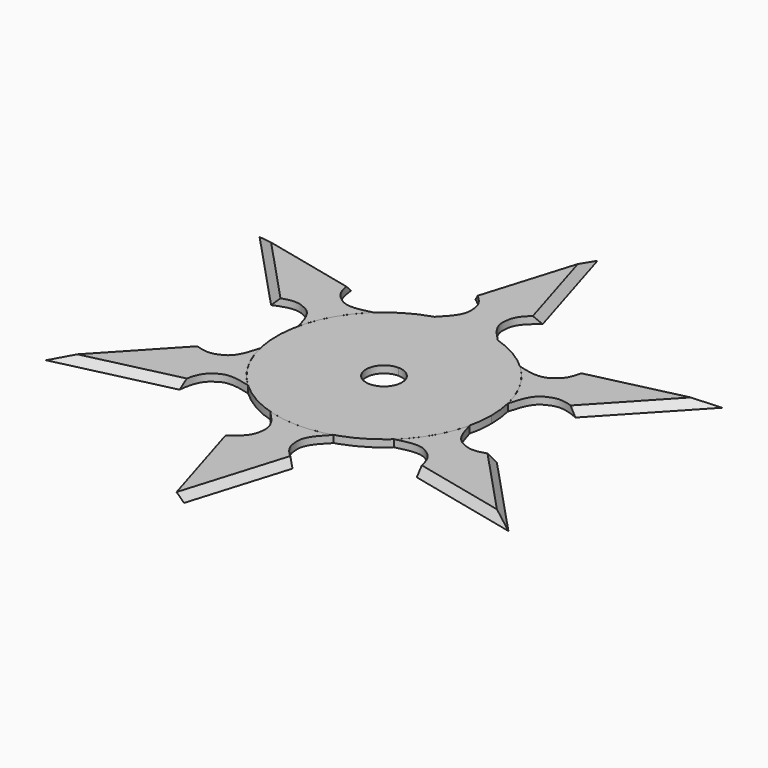
from build123d import *

# Parameters (mm, degrees)
F1_DEPTH      = 1.27
F2_COUNT      = 6
F3_DEPTH      = 1.27
F4_T1_DEPTH   = 28.2648616639
F4_T3_DEPTH   = 28.2648616639
F4_2_T1_DEPTH = 28.2648616639
F4_2_T3_DEPTH = 28.2648616639
F4_3_T1_DEPTH = 28.2648616639
F4_3_T3_DEPTH = 28.2648616639
F4_4_T1_DEPTH = 28.2648616639
F4_4_T3_DEPTH = 28.2648616639
F4_5_T1_DEPTH = 28.2648616639
F4_5_T3_DEPTH = 28.2648616639
F4_6_T1_DEPTH = 28.2648616639
F4_6_T3_DEPTH = 28.2648616639


# Not quite as in the source:
# - a fillet or chamfer that OpenCascade refuses, or shapes differently, is made with other operations: its cross-section is extruded or revolved along the edge and cut away or added


with BuildPart() as f1:
    # F0 (on Top) → F1 (new body)
    with BuildSketch(Plane.XY):
        Polygon((0, 27.8319306672), (6.0893329792, 27.8319306672), (0, 47.8763319552), align=None)
        Polygon((0, 47.8763319552), (-6.0893329792, 27.8319306672), (0, 27.8319306672), align=None)
        with BuildLine():
            add(Edge.make_bspline(
                [(-5.6085209245, 18.2056857338), (-2.7667914864, 20.9939918215), (-2.759898495, 23.1821026248), (-3.1363011766, 25.7094376402), (-6.0893329792, 27.8319306672)],
                knots=[0, 0, 0, 0, 0.5044710626, 1, 1, 1, 1], degree=3))
            ThreePointArc((-5.6085209245, 18.2056857338), (-2.8358584917, 18.8377388934), (0, 19.05))
            Line((0, 19.05), (0, 27.8319306672))
            Line((0, 27.8319306672), (-6.0893329792, 27.8319306672))
        make_face()
        with BuildLine():
            ThreePointArc((0, 19.05), (2.8358584917, 18.8377388934), (5.6085209245, 18.2056857338))
            add(Edge.make_bspline(
                [(5.6085209245, 18.2056857338), (2.7667914864, 20.9939918215), (2.759898495, 23.1821026248), (3.1363011766, 25.7094376402), (6.0893329792, 27.8319306672)],
                knots=[0, 0, 0, 0, 0.5044710626, 1, 1, 1, 1], degree=3))
            Line((6.0893329792, 27.8319306672), (0, 27.8319306672))
            Line((0, 27.8319306672), (0, 19.05))
        make_face()
    extrude(amount=F1_DEPTH)


with BuildPart() as f2_1:
    # F2: instance of F1
    add(f1.part.rotate(Axis((0, 0, 0), (0, 0, 1)), 1 * 360 / F2_COUNT))

    # F4#2: chamfer of 1.4224 on 2 edges, made by hand

    # F4_2_s2 → F4_2_t1 (cut)
    with BuildSketch(Plane(origin=(-20.6503164596, 4.8060973638, 0), x_dir=(0, 0, 1), z_dir=(-0.9739695304, 0.2266789665, 0))):
        Polygon((-0.1524, 13.9164538313), (1.27, 12.4940538313), (1.27, 13.9164538313), align=None)
    extrude(amount=F4_2_T1_DEPTH, mode=Mode.SUBTRACT)

    # F4_2_s4 → F4_2_t3 (cut)
    with BuildSketch(Plane(origin=(-33.8005854034, 36.1180372572, 0), x_dir=(0, 0, 1), z_dir=(0.6832945087, -0.7301428726, 0))):
        Polygon((-0.1524, 13.9164538313), (1.27, 12.4940538313), (1.27, 13.9164538313), align=None)
    extrude(amount=F4_2_T3_DEPTH, mode=Mode.SUBTRACT)


with BuildPart() as f2_2:
    # F2: instance of F1
    add(f1.part.rotate(Axis((0, 0, 0), (0, 0, 1)), 2 * 360 / F2_COUNT))

    # F4#3: chamfer of 1.4224 on 2 edges, made by hand

    # F4_3_s2 → F4_3_t1 (cut)
    with BuildSketch(Plane(origin=(-48.1794305013, -11.2131469935, 0), x_dir=(0, 0, 1), z_dir=(0.9739695304, 0.2266789665, 0))):
        Polygon((-0.1524, 13.9164538313), (1.27, 12.4940538313), (1.27, 13.9164538313), align=None)
    extrude(amount=F4_3_T1_DEPTH, mode=Mode.SUBTRACT)

    # F4_3_s4 → F4_3_t3 (cut)
    with BuildSketch(Plane(origin=(-14.4873606399, -15.4806499682, 0), x_dir=(0, 0, 1), z_dir=(-0.6832945087, -0.7301428726, 0))):
        Polygon((-0.1524, 13.9164538313), (1.27, 12.4940538313), (1.27, 13.9164538313), align=None)
    extrude(amount=F4_3_T3_DEPTH, mode=Mode.SUBTRACT)


with BuildPart() as f2_3:
    # F2: instance of F1
    add(f1.part.rotate(Axis((0, 0, 0), (0, 0, 1)), 3 * 360 / F2_COUNT))

    # F4#4: chamfer of 1.4224 on 2 edges, made by hand

    # F4_4_s2 → F4_4_t1 (cut)
    with BuildSketch(Plane(origin=(-14.3788450979, -47.3311842507, 0), x_dir=(0, 0, 1), z_dir=(0.2906750217, 0.9568218391, 0))):
        Polygon((-0.1524, 13.9164538313), (1.27, 12.4940538313), (1.27, 13.9164538313), align=None)
    extrude(amount=F4_4_T1_DEPTH, mode=Mode.SUBTRACT)

    # F4_4_s4 → F4_4_t3 (cut)
    with BuildSketch(Plane(origin=(6.1629558196, -20.2867473321, 0), x_dir=(0, 0, 1), z_dir=(0.2906750217, -0.9568218391, 0))):
        Polygon((1.4224, 13.9164538313), (0, 12.4940538313), (0, 13.9164538313), align=None)
    extrude(amount=F4_4_T3_DEPTH, mode=Mode.SUBTRACT)


with BuildPart() as f2_4:
    # F2: instance of F1
    add(f1.part.rotate(Axis((0, 0, 0), (0, 0, 1)), 4 * 360 / F2_COUNT))

    # F4#5: chamfer of 1.4224 on 2 edges, made by hand

    # F4_5_s2 → F4_5_t1 (cut)
    with BuildSketch(Plane(origin=(33.8005854034, -36.1180372572, 0), x_dir=(0, 0, 1), z_dir=(-0.6832945087, 0.7301428726, 0))):
        Polygon((-0.1524, 13.9164538313), (1.27, 12.4940538313), (1.27, 13.9164538313), align=None)
    extrude(amount=F4_5_T1_DEPTH, mode=Mode.SUBTRACT)

    # F4_5_s4 → F4_5_t3 (cut)
    with BuildSketch(Plane(origin=(20.6503164596, -4.8060973638, 0), x_dir=(0, 0, 1), z_dir=(0.9739695304, -0.2266789665, 0))):
        Polygon((-0.1524, 13.9164538313), (1.27, 12.4940538313), (1.27, 13.9164538313), align=None)
    extrude(amount=F4_5_T3_DEPTH, mode=Mode.SUBTRACT)


with BuildPart() as f2_5:
    # F2: instance of F1
    add(f1.part.rotate(Axis((0, 0, 0), (0, 0, 1)), 5 * 360 / F2_COUNT))

    # F4#6: chamfer of 1.4224 on 2 edges, made by hand

    # F4_6_s2 → F4_6_t1 (cut)
    with BuildSketch(Plane(origin=(48.1794305013, 11.2131469935, 0), x_dir=(0, 0, 1), z_dir=(-0.9739695304, -0.2266789665, 0))):
        Polygon((-0.1524, 13.9164538313), (1.27, 12.4940538313), (1.27, 13.9164538313), align=None)
    extrude(amount=F4_6_T1_DEPTH, mode=Mode.SUBTRACT)

    # F4_6_s4 → F4_6_t3 (cut)
    with BuildSketch(Plane(origin=(14.4873606399, 15.4806499682, 0), x_dir=(0, 0, 1), z_dir=(0.6832945087, 0.7301428726, 0))):
        Polygon((-0.1524, 13.9164538313), (1.27, 12.4940538313), (1.27, 13.9164538313), align=None)
    extrude(amount=F4_6_T3_DEPTH, mode=Mode.SUBTRACT)


with BuildPart() as f1_1:
    add(f1.part)

    # F0 (on Top) → F3 (join)
    with BuildSketch(Plane.XY):
        with BuildLine():
            ThreePointArc((-5.6085209245, 18.2056857338), (-11.3150381437, -15.3255476837), (19.05, 0))
            ThreePointArc((19.05, 0), (15.3255476837, 11.3150381437), (5.6085209245, 18.2056857338))
            ThreePointArc((5.6085209245, 18.2056857338), (2.8358584917, 18.8377388934), (0, 19.05))
            ThreePointArc((0, 19.05), (-2.8358584917, 18.8377388934), (-5.6085209245, 18.2056857338))
        make_face()
        with BuildLine():
            ThreePointArc((3.175, 0), (-2.2450640303, -2.2450640303), (0, 3.175))
            ThreePointArc((0, 3.175), (2.2450640303, 2.2450640303), (3.175, 0))
        make_face(mode=Mode.SUBTRACT)
    extrude(amount=F3_DEPTH)

    # F4: chamfer of 1.4224 on 2 edges, made by hand

    # F4_s2 → F4_t1 (cut)
    with BuildSketch(Plane(origin=(14.3788450979, 47.3311842507, 0), x_dir=(0, 0, 1), z_dir=(-0.2906750217, -0.9568218391, 0))):
        Polygon((-0.1524, 13.9164538313), (1.27, 12.4940538313), (1.27, 13.9164538313), align=None)
    extrude(amount=F4_T1_DEPTH, mode=Mode.SUBTRACT)

    # F4_s4 → F4_t3 (cut)
    with BuildSketch(Plane(origin=(-6.1629558196, 20.2867473321, 0), x_dir=(0, 0, 1), z_dir=(-0.2906750217, 0.9568218391, 0))):
        Polygon((-0.1524, 13.9164538313), (1.27, 12.4940538313), (1.27, 13.9164538313), align=None)
    extrude(amount=F4_T3_DEPTH, mode=Mode.SUBTRACT)


solid = Compound([f2_1.part, f2_2.part, f2_3.part, f2_4.part, f2_5.part, f1_1.part])
